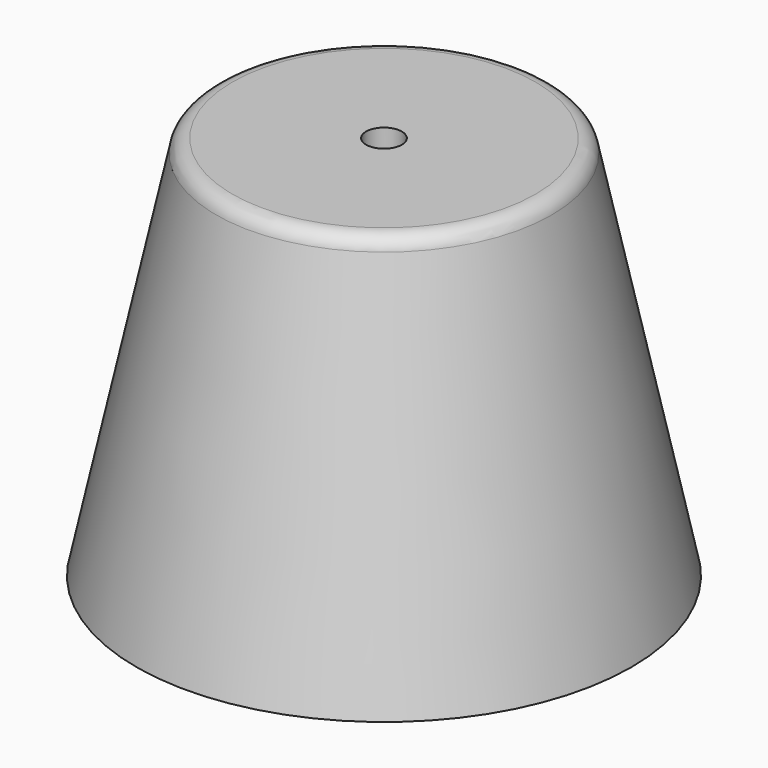
from build123d import *

# Parameters (mm, degrees)
F1_R     = 45
F2_R     = 30
F4_T     = -0.8
F5_R     = 7.5
F6_DEPTH = 10
F7_R     = 3.25
F8_DEPTH = 10.8010001
F9_R     = 3


with BuildPart() as f3:
    # F1 (on Top) → F3 section 0
    with BuildSketch(Plane.XY):
        Circle(F1_R)
    # F2 (on offset) → F3 section 1
    with BuildSketch(Plane.XY.offset(70)):
        Circle(F2_R)
    loft()

    # F4
    f4_openings = [f3.faces().sort_by_distance(p)[0] for p in [
        (0, 0, 0),
    ]]
    offset(amount=F4_T, openings=f4_openings, kind=Kind.INTERSECTION)

    # F5 (on face) → F6 (join)
    with BuildSketch(Plane(origin=(0, 0, 69.2), x_dir=(1, 0, 0), z_dir=(0, 0, -1))):
        Circle(F5_R)
    extrude(amount=F6_DEPTH)

    # F7 (on face) → F8 (cut, through all)
    with BuildSketch(Plane(origin=(0, 0, 59.2), x_dir=(1, 0, 0), z_dir=(0, 0, -1))):
        Circle(F7_R)
    extrude(amount=-F8_DEPTH, mode=Mode.SUBTRACT)

    # F9
    f9_edges = [f3.edges().sort_by_distance(p)[0] for p in [
        (-30, 0, 70),
    ]]
    fillet(f9_edges, radius=F9_R)


solid = f3.part
